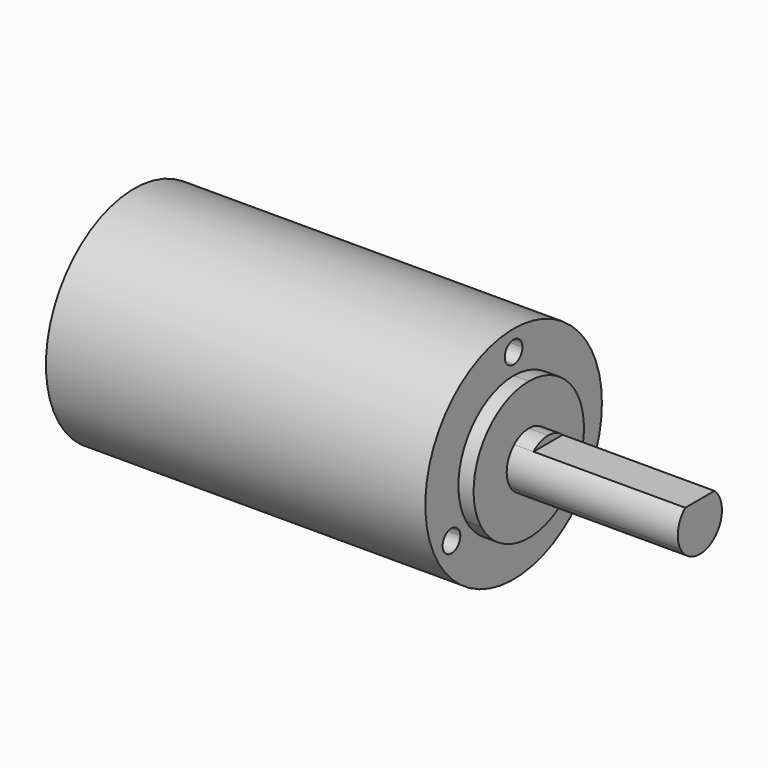
from build123d import *

# Parameters (mm, degrees)
F1_DEPTH = 13.5
F2_DEPTH = 1.1
F0_R     = 8
F3_DEPTH = 27.5
F6_DEPTH = 20
F7_DEPTH = 2.5


# Not quite as in the source:
# - a feature of the source that left no trace in its solid (it failed there, or was rolled back) is left out


with BuildPart() as f1:
    # F0 (on Right) → F1 (new body)
    with BuildSketch(Plane.YZ):
        with BuildLine():
            ThreePointArc((-1.3228756555, 1.5), (-1.9737385652, 0.323041911), (-1.7320508076, -1))
            Line((-1.7320508076, -1), (0, 0))
            Line((0, 0), (0, 1.5))
            Line((0, 1.5), (-1.3228756555, 1.5))
        make_face()
        with BuildLine():
            Line((0, 0), (1.7320508076, -1))
            ThreePointArc((1.7320508076, -1), (1.9318516526, -0.5176380902), (2, 0))
            ThreePointArc((2, 0), (1.8228756555, 0.8228756555), (1.3228756555, 1.5))
            Line((1.3228756555, 1.5), (0, 1.5))
            Line((0, 1.5), (0, 0))
        make_face()
        with BuildLine():
            ThreePointArc((-1.7320508076, -1), (0, -2), (1.7320508076, -1))
            Line((1.7320508076, -1), (0, 0))
            Line((0, 0), (-1.7320508076, -1))
        make_face()
    extrude(amount=F1_DEPTH)

    # F0 (on Right) → F2 (join)
    with BuildSketch(Plane.YZ):
        with BuildLine():
            Line((0, 2), (0, 5))
            ThreePointArc((0, 5), (-4.3301270189, 2.5), (-4.3301270189, -2.5))
            Line((-4.3301270189, -2.5), (-1.7320508076, -1))
            ThreePointArc((-1.7320508076, -1), (-1.9737385652, 0.323041911), (-1.3228756555, 1.5))
            ThreePointArc((-1.3228756555, 1.5), (-0.7071067812, 1.8708286934), (0, 2))
        make_face()
        with BuildLine():
            ThreePointArc((-4.3301270189, -2.5), (0, -5), (4.3301270189, -2.5))
            Line((4.3301270189, -2.5), (1.7320508076, -1))
            ThreePointArc((1.7320508076, -1), (0, -2), (-1.7320508076, -1))
            Line((-1.7320508076, -1), (-4.3301270189, -2.5))
        make_face()
        with BuildLine():
            ThreePointArc((4.3301270189, -2.5), (4.8296291314, -1.2940952255), (5, 0))
            ThreePointArc((5, 0), (3.5355339059, 3.5355339059), (0, 5))
            Line((0, 5), (0, 2))
            ThreePointArc((0, 2), (0.7071067812, 1.8708286934), (1.3228756555, 1.5))
            ThreePointArc((1.3228756555, 1.5), (1.8228756555, 0.8228756555), (2, 0))
            ThreePointArc((2, 0), (1.9318516526, -0.5176380902), (1.7320508076, -1))
            Line((1.7320508076, -1), (4.3301270189, -2.5))
        make_face()
    extrude(amount=F2_DEPTH)


with BuildPart() as f3:
    # F0 (on Right) → F3 (new body)
    with BuildSketch(Plane.YZ):
        Circle(F0_R)
        with BuildLine():
            ThreePointArc((-4.8291651246, -3.25), (-6.4019057856, -3.4570552361), (-4.9363448016, -2.85))
            ThreePointArc((-4.9363448016, -2.85), (-4.8564244636, -3.0429447639), (-4.8291651246, -3.25))
        make_face(mode=Mode.SUBTRACT)
        with BuildLine():
            ThreePointArc((6.4291651246, -3.25), (5.4221098885, -4.022740661), (4.9363448016, -2.85))
            ThreePointArc((4.9363448016, -2.85), (5.8362203607, -2.477259339), (6.4291651246, -3.25))
        make_face(mode=Mode.SUBTRACT)
        with BuildLine():
            ThreePointArc((0, 5), (3.5355339059, 3.5355339059), (5, 0))
            ThreePointArc((5, 0), (4.8296291314, -1.2940952255), (4.3301270189, -2.5))
            ThreePointArc((4.3301270189, -2.5), (0, -5), (-4.3301270189, -2.5))
            ThreePointArc((-4.3301270189, -2.5), (-4.3301270189, 2.5), (0, 5))
        make_face(mode=Mode.SUBTRACT)
        with BuildLine():
            ThreePointArc((0.8, 6.5), (0.5656854249, 5.9343145751), (0, 5.7))
            ThreePointArc((0, 5.7), (-0.5656854249, 7.0656854249), (0.8, 6.5))
        make_face(mode=Mode.SUBTRACT)
        with BuildLine():
            ThreePointArc((-4.3301270189, -2.5), (0, -5), (4.3301270189, -2.5))
            Line((4.3301270189, -2.5), (1.7320508076, -1))
            ThreePointArc((1.7320508076, -1), (0, -2), (-1.7320508076, -1))
            Line((-1.7320508076, -1), (-4.3301270189, -2.5))
        make_face()
    extrude(amount=-F3_DEPTH)

    # F4 (on face) → F6 (cut)
    with BuildSketch(Plane(origin=(-27.5, 0, 0), x_dir=(0, -1, 0), z_dir=(-1, 0, 0))):
        with BuildLine():
            ThreePointArc((-3.7455598714, -2.1625), (-4.1335062489, -1.8542715177), (-4.6273989915, -1.8939848399))
            ThreePointArc((-4.6273989915, -1.8939848399), (-4.4890011863, -2.2020146116), (-4.3301270189, -2.5))
            Line((-4.3301270189, -2.5), (-3.7455598714, -2.1625))
        make_face()
        with BuildLine():
            ThreePointArc((-4.3301270189, -2.5), (-4.4890011863, -2.2020146116), (-4.6273989915, -1.8939848399))
            ThreePointArc((-4.6273989915, -1.8939848399), (-4.6871749278, -3.0728366178), (-3.6551270189, -2.5))
            ThreePointArc((-3.6551270189, -2.5), (-3.6781270862, -2.3252971446), (-3.7455598714, -2.1625))
            Line((-3.7455598714, -2.1625), (-4.3301270189, -2.5))
        make_face()
        with BuildLine():
            ThreePointArc((0.67346051, 4.9544375), (0, 5), (-0.67346051, 4.9544375))
            ThreePointArc((-0.67346051, 4.9544375), (0, 4.325), (0.67346051, 4.9544375))
        make_face()
        with BuildLine():
            ThreePointArc((0.67346051, 4.9544375), (0.6746150177, 4.9772057494), (0.675, 5))
            ThreePointArc((0.675, 5), (-0.0227942506, 5.6746150177), (-0.67346051, 4.9544375))
            ThreePointArc((-0.67346051, 4.9544375), (0, 5), (0.67346051, 4.9544375))
        make_face()
        with BuildLine():
            ThreePointArc((4.3301270189, -2.5), (4.4890011863, -2.2020146116), (4.6273989915, -1.8939848399))
            ThreePointArc((4.6273989915, -1.8939848399), (4.1335062489, -1.8542715177), (3.7455598714, -2.1625))
            Line((3.7455598714, -2.1625), (4.3301270189, -2.5))
        make_face()
        with BuildLine():
            ThreePointArc((5.0051270189, -2.5), (4.9029636368, -2.1429520911), (4.6273989915, -1.8939848399))
            ThreePointArc((4.6273989915, -1.8939848399), (4.4890011863, -2.2020146116), (4.3301270189, -2.5))
            Line((4.3301270189, -2.5), (3.7455598714, -2.1625))
            ThreePointArc((3.7455598714, -2.1625), (4.1554241635, -3.1519999327), (5.0051270189, -2.5))
        make_face()
    extrude(amount=-F6_DEPTH, mode=Mode.SUBTRACT)


with BuildPart() as f3b:
    # F0 (on Right) → F3, piece 2 (new body)
    with BuildSketch(Plane.YZ):
        with BuildLine():
            Line((0, 1.5), (0, 2))
            ThreePointArc((0, 2), (-0.7071067812, 1.8708286934), (-1.3228756555, 1.5))
            Line((-1.3228756555, 1.5), (0, 1.5))
        make_face()
        with BuildLine():
            ThreePointArc((1.3228756555, 1.5), (0.7071067812, 1.8708286934), (0, 2))
            Line((0, 2), (0, 1.5))
            Line((0, 1.5), (1.3228756555, 1.5))
        make_face()
        with BuildLine():
            Line((0, 0), (1.7320508076, -1))
            ThreePointArc((1.7320508076, -1), (1.9318516526, -0.5176380902), (2, 0))
            ThreePointArc((2, 0), (1.8228756555, 0.8228756555), (1.3228756555, 1.5))
            Line((1.3228756555, 1.5), (0, 1.5))
            Line((0, 1.5), (0, 0))
        make_face()
        with BuildLine():
            ThreePointArc((-1.3228756555, 1.5), (-1.9737385652, 0.323041911), (-1.7320508076, -1))
            Line((-1.7320508076, -1), (0, 0))
            Line((0, 0), (0, 1.5))
            Line((0, 1.5), (-1.3228756555, 1.5))
        make_face()
    extrude(amount=-F3_DEPTH)


with BuildPart() as f7:
    # F0 (on Right) → F7 (new body)
    with BuildSketch(Plane.YZ):
        with BuildLine():
            Line((0, 1.5), (0, 2))
            ThreePointArc((0, 2), (-0.7071067812, 1.8708286934), (-1.3228756555, 1.5))
            Line((-1.3228756555, 1.5), (0, 1.5))
        make_face()
        with BuildLine():
            ThreePointArc((1.3228756555, 1.5), (0.7071067812, 1.8708286934), (0, 2))
            Line((0, 2), (0, 1.5))
            Line((0, 1.5), (1.3228756555, 1.5))
        make_face()
    extrude(amount=F7_DEPTH)


solid = Compound([f1.part, f3.part, f3b.part, f7.part])
